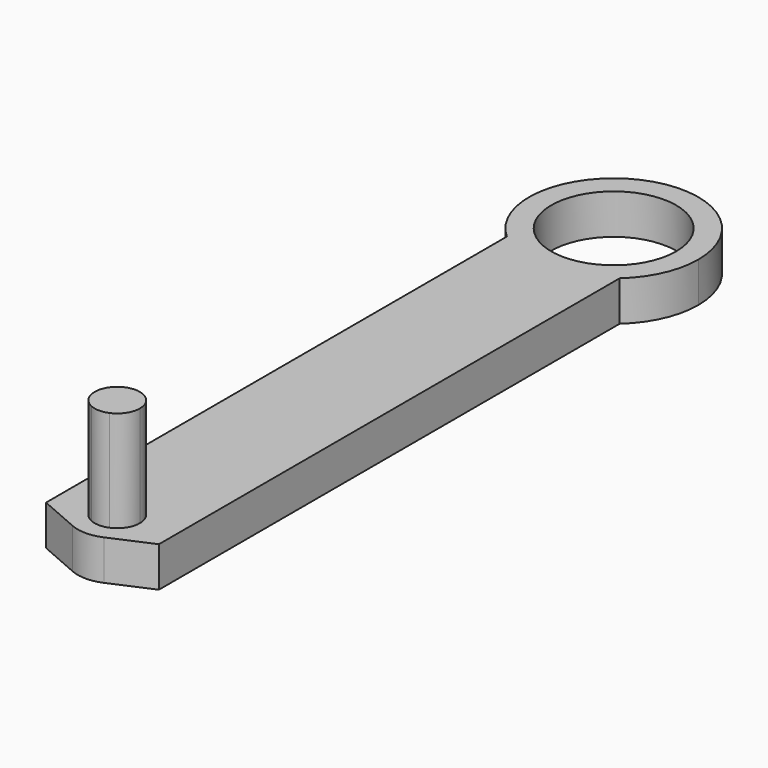
from build123d import *

# Parameters (mm, degrees)
F1_DEPTH = 7.1
F2_DEPTH = 25


with BuildPart() as f1:
    # F0 (on Top) → F1 (new body)
    with BuildSketch(Plane.XY):
        with BuildLine():
            Line((-2.752413094, -69.1138580441), (1.247586906, -69.1138580441))
            Line((1.247586906, -69.1138580441), (5.247586906, -69.1138580441))
            ThreePointArc((5.247586906, -69.1138580441), (1.247586906, -65.1138580441), (-2.752413094, -69.1138580441))
        make_face()
        with BuildLine():
            Line((5.247586906, -69.1138580441), (1.247586906, -69.1138580441))
            Line((1.247586906, -69.1138580441), (-2.752413094, -69.1138580441))
            ThreePointArc((-2.752413094, -69.1138580441), (-2.0990532002, -71.3047482742), (-0.352413094, -72.7799186001))
            ThreePointArc((-0.352413094, -72.7799186001), (1.247586906, -73.1138580441), (2.847586906, -72.7799186001))
            ThreePointArc((2.847586906, -72.7799186001), (4.5942270121, -71.3047482742), (5.247586906, -69.1138580441))
        make_face()
        with BuildLine():
            ThreePointArc((-2.752413094, -69.1138580441), (1.247586906, -65.1138580441), (5.247586906, -69.1138580441))
            Line((5.247586906, -69.1138580441), (8.247586906, -69.1138580441))
            ThreePointArc((8.247586906, -69.1138580441), (1.247586906, -62.1138580441), (-5.752413094, -69.1138580441))
            Line((-5.752413094, -69.1138580441), (-2.752413094, -69.1138580441))
        make_face()
        with BuildLine():
            Line((8.247586906, -69.1138580441), (5.247586906, -69.1138580441))
            ThreePointArc((5.247586906, -69.1138580441), (4.5942270121, -71.3047482742), (2.847586906, -72.7799186001))
            Line((2.847586906, -72.7799186001), (8.1125655384, -70.4820935415))
            ThreePointArc((8.1125655384, -70.4820935415), (8.2137497819, -69.8012987954), (8.247586906, -69.1138580441))
        make_face()
        with BuildLine():
            ThreePointArc((-0.352413094, -72.7799186001), (-2.0990532002, -71.3047482742), (-2.752413094, -69.1138580441))
            Line((-2.752413094, -69.1138580441), (-5.752413094, -69.1138580441))
            ThreePointArc((-5.752413094, -69.1138580441), (-5.7185759699, -69.8012987954), (-5.6173917265, -70.4820935415))
            Line((-5.6173917265, -70.4820935415), (-0.352413094, -72.7799186001))
        make_face()
        with BuildLine():
            ThreePointArc((-5.752413094, -69.1138580441), (1.247586906, -62.1138580441), (8.247586906, -69.1138580441))
            Line((8.247586906, -69.1138580441), (11.247586906, -69.1138580441))
            Line((11.247586906, -69.1138580441), (11.247586906, 29.7058020684))
            ThreePointArc((11.247586906, 29.7058020684), (1.247586906, 25.8861419559), (-8.752413094, 29.7058020684))
            Line((-8.752413094, 29.7058020684), (-8.752413094, -69.1138580441))
            Line((-8.752413094, -69.1138580441), (-5.752413094, -69.1138580441))
        make_face()
        with BuildLine():
            Line((11.247586906, -69.1138580441), (8.247586906, -69.1138580441))
            ThreePointArc((8.247586906, -69.1138580441), (8.2137497819, -69.8012987954), (8.1125655384, -70.4820935415))
            Line((8.1125655384, -70.4820935415), (11.247586906, -69.1138580441))
        make_face()
        with BuildLine():
            Line((8.1125655384, -70.4820935415), (2.847586906, -72.7799186001))
            ThreePointArc((2.847586906, -72.7799186001), (1.247586906, -73.1138580441), (-0.352413094, -72.7799186001))
            Line((-0.352413094, -72.7799186001), (-5.6173917265, -70.4820935415))
            ThreePointArc((-5.6173917265, -70.4820935415), (-4.2041963042, -73.5045367877), (-1.552413094, -75.5294640171))
            ThreePointArc((-1.552413094, -75.5294640171), (1.247586906, -76.1138580441), (4.047586906, -75.5294640171))
            ThreePointArc((4.047586906, -75.5294640171), (6.6993701161, -73.5045367877), (8.1125655384, -70.4820935415))
        make_face()
        with BuildLine():
            ThreePointArc((-5.6173917265, -70.4820935415), (-5.7185759699, -69.8012987954), (-5.752413094, -69.1138580441))
            Line((-5.752413094, -69.1138580441), (-8.752413094, -69.1138580441))
            Line((-8.752413094, -69.1138580441), (-5.6173917265, -70.4820935415))
        make_face()
        with BuildLine():
            Line((11.247586906, -72.3871263977), (11.247586906, -69.1138580441))
            Line((11.247586906, -69.1138580441), (8.1125655384, -70.4820935415))
            ThreePointArc((8.1125655384, -70.4820935415), (6.6993701161, -73.5045367877), (4.047586906, -75.5294640171))
            Line((4.047586906, -75.5294640171), (11.247586906, -72.3871263977))
        make_face()
        with BuildLine():
            Line((-5.6173917265, -70.4820935415), (-8.752413094, -69.1138580441))
            Line((-8.752413094, -69.1138580441), (-8.752413094, -72.3871263977))
            Line((-8.752413094, -72.3871263977), (-1.552413094, -75.5294640171))
            ThreePointArc((-1.552413094, -75.5294640171), (-4.2041963042, -73.5045367877), (-5.6173917265, -70.4820935415))
        make_face()
        with BuildLine():
            ThreePointArc((-8.752413094, 29.7058020684), (1.247586906, 25.8861419559), (11.247586906, 29.7058020684))
            Line((11.247586906, 29.7058020684), (11.247586906, 36.1263494184))
            ThreePointArc((11.247586906, 36.1263494184), (1.247586906, 29.8111419559), (-8.752413094, 36.1263494184))
            Line((-8.752413094, 36.1263494184), (-8.752413094, 29.7058020684))
        make_face()
        with BuildLine():
            Line((11.247586906, 36.1263494184), (11.247586906, 29.7058020684))
            ThreePointArc((11.247586906, 29.7058020684), (14.9406508436, 34.7624175989), (16.247586906, 40.8861419559))
            ThreePointArc((16.247586906, 40.8861419559), (-4.876137451, 54.5792058935), (-8.752413094, 29.7058020684))
            Line((-8.752413094, 29.7058020684), (-8.752413094, 36.1263494184))
            ThreePointArc((-8.752413094, 36.1263494184), (-1.1922517158, 51.6890495506), (12.322586906, 40.8861419559))
            ThreePointArc((12.322586906, 40.8861419559), (12.0504945007, 38.4463033341), (11.247586906, 36.1263494184))
        make_face()
    extrude(amount=F1_DEPTH)

    # F0 (on Top) → F2 (join)
    with BuildSketch(Plane.XY):
        with BuildLine():
            Line((-2.752413094, -69.1138580441), (1.247586906, -69.1138580441))
            Line((1.247586906, -69.1138580441), (5.247586906, -69.1138580441))
            ThreePointArc((5.247586906, -69.1138580441), (1.247586906, -65.1138580441), (-2.752413094, -69.1138580441))
        make_face()
        with BuildLine():
            Line((5.247586906, -69.1138580441), (1.247586906, -69.1138580441))
            Line((1.247586906, -69.1138580441), (-2.752413094, -69.1138580441))
            ThreePointArc((-2.752413094, -69.1138580441), (-2.0990532002, -71.3047482742), (-0.352413094, -72.7799186001))
            ThreePointArc((-0.352413094, -72.7799186001), (1.247586906, -73.1138580441), (2.847586906, -72.7799186001))
            ThreePointArc((2.847586906, -72.7799186001), (4.5942270121, -71.3047482742), (5.247586906, -69.1138580441))
        make_face()
    extrude(amount=F2_DEPTH)


solid = f1.part
